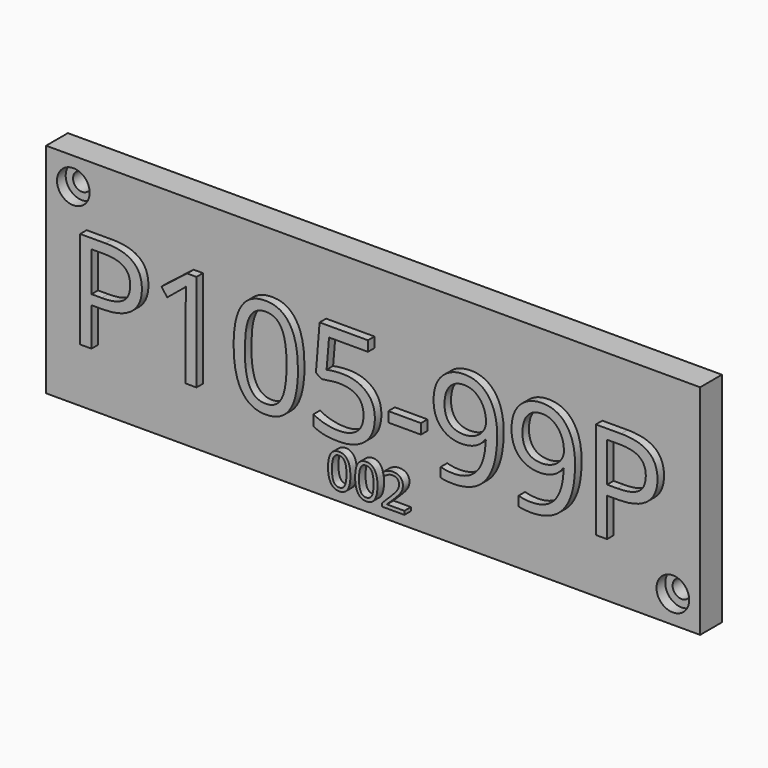
from build123d import *

# Parameters (mm, degrees)
F0_W           = 120
F0_H           = 40
F1_DEPTH       = 5
F3_D           = 3.3
F3_CBORE_D     = 6
F3_CBORE_DEPTH = 2
F4_TEXT_SIZE   = 25.0115465236
F5_DEPTH       = 1.5
F6_TEXT_SIZE   = 8.6885691013
F7_DEPTH       = 1.5


# Not quite as in the source:
# - Text() gives the source's letters only with a copy of the font that has no kerning and outlines rounded to 1/6400 em; it was checked with that copy


with BuildPart() as f1:
    # F0 (on Front) → F1 (new body)
    with BuildSketch(Plane.XZ):
        Rectangle(F0_W, F0_H)
    extrude(amount=F1_DEPTH)

    # F3 (through all)
    with Locations(Plane.XZ.offset(5)):
        with Locations((-55, 15), (55, -15)):
            CounterBoreHole(F3_D / 2, F3_CBORE_D / 2, F3_CBORE_DEPTH)

    # F4 (on face) → F5 (join)
    with BuildSketch(Plane.XZ.offset(5)):
        with Locations((-55, -9.0817786795)):
            Text('P105-99P', F4_TEXT_SIZE, font='Open Sans', text_align=(TextAlign.LEFT, TextAlign.BOTTOM))
    extrude(amount=F5_DEPTH)

    # F6 (on face) → F7 (join)
    with BuildSketch(Plane.XZ.offset(5)):
        with Locations((-7.5, -17.2557697529)):
            Text('002', F6_TEXT_SIZE, font='Open Sans', text_align=(TextAlign.LEFT, TextAlign.BOTTOM))
    extrude(amount=F7_DEPTH)


solid = f1.part
